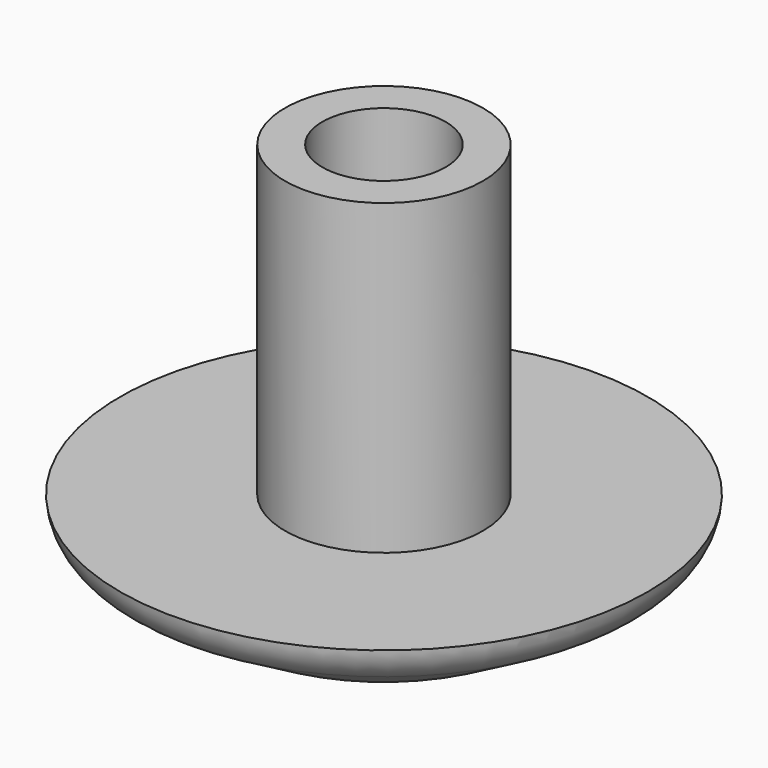
from build123d import *

# Parameters (mm, degrees)
F0_R     = 6
F1_DEPTH = 2
F2_SIZE2 = 2.5980762114
F2_SIZE  = 1.5
F4_R     = 2.25
F4_R_2   = 1.4
F5_DEPTH = 7
F6_R     = 1.2


# Not quite as in the source:
# - a fillet or chamfer that OpenCascade refuses, or shapes differently, is made with other operations: its cross-section is extruded or revolved along the edge and cut away or added


with BuildPart() as f1:
    # F0 (on Top) → F1 (new body)
    with BuildSketch(Plane.XY):
        Circle(F0_R)
    extrude(amount=F1_DEPTH)

    # F2
    f2_edges = [f1.edges().sort_by_distance(p)[0] for p in [
        (-6, 0, 0),
    ]]
    f2_side = f1.faces().sort_by_distance((-6, 0, 1))[0]
    chamfer(f2_edges, length=F2_SIZE, length2=F2_SIZE2, reference=f2_side)

    # F3: fillet of radius 1 on 2 edges, made by hand

    # F3_s1 → F3_t2 (revolve, cut)
    with BuildSketch(Plane.XZ):
        with BuildLine():
            ThreePointArc((3.6339745962, 0.1339745962), (3.3927936413, 0.0340741737), (3.1339745962, 0))
            Line((3.1339745962, 0), (3.4019237886, 0))
            Line((3.4019237886, 0), (3.6339745962, 0.1339745962))
        make_face()
    revolve(axis=Axis((0, 0, 0), (0, 0, 1)), mode=Mode.SUBTRACT)

    # F3_s3 → F3_t4 (revolve, cut)
    with BuildSketch(Plane.XZ):
        with BuildLine():
            ThreePointArc((6, 2), (5.8486778537, 1.5452494356), (5.5031382462, 1.2131367327))
            Line((5.5031382462, 1.2131367327), (6, 1.5))
            Line((6, 1.5), (6, 2))
        make_face()
    revolve(axis=Axis((0, 0, 1.5), (0, 0, 1)), mode=Mode.SUBTRACT)

    # F4 (on face) → F5 (join)
    with BuildSketch(Plane.XY.offset(2)):
        Circle(F4_R)
        Circle(F4_R_2, mode=Mode.SUBTRACT)
    extrude(amount=F5_DEPTH)

    # F6
    f6_edges = [f1.edges().sort_by_distance(p)[0] for p in [
        (-1.4, 0, 2),
    ]]
    fillet(f6_edges, radius=F6_R)


solid = f1.part
